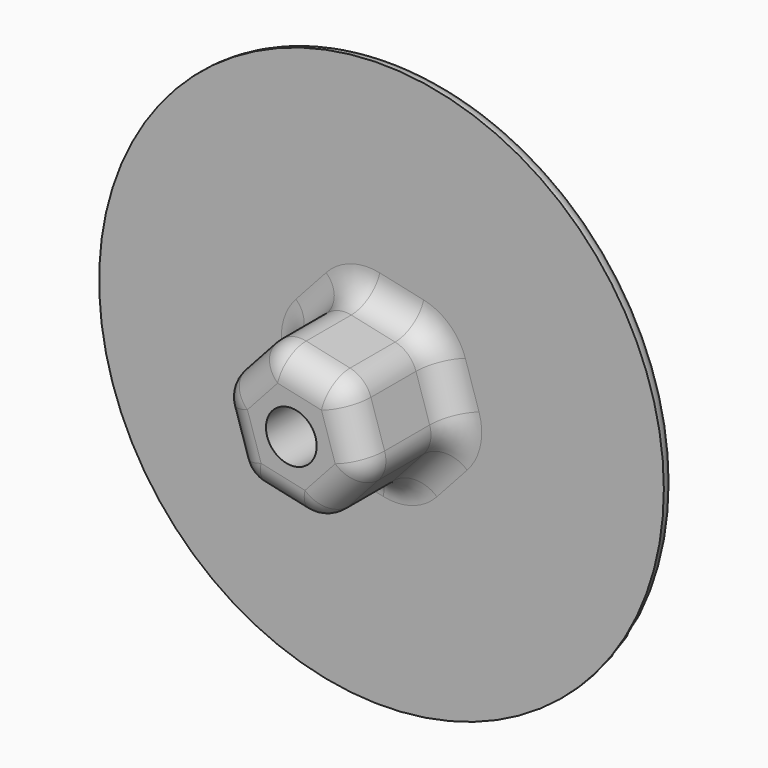
from build123d import *

# Parameters (mm, degrees)
F0_R     = 50.1
F0_R_2   = 4.5
F1_DEPTH = 3
F2_R     = 4.5
F3_DEPTH = 20
F4_R     = 2.99999
F5_R     = 5
F6_R     = 5


# Not quite as in the source:
# - a fillet or chamfer is up to 0.001 mm smaller than in the source, because OpenCascade refuses the exact size


with BuildPart() as f1:
    # F0 (on Front) → F1 (new body)
    with BuildSketch(Plane.XZ):
        Circle(F0_R)
        Circle(F0_R_2, mode=Mode.SUBTRACT)
    extrude(amount=F1_DEPTH)

    # F2 (on face) → F3 (join)
    with BuildSketch(Plane.XZ.offset(3)):
        Polygon((9.2398859849, 10.167053197), (-4.1849833578, 13.0855025895), (-13.4248693427, 2.9184493925), (-9.2398859849, -10.167053197), (4.1849833578, -13.0855025895), (13.4248693427, -2.9184493925), align=None)
        Circle(F2_R, mode=Mode.SUBTRACT)
    extrude(amount=F3_DEPTH)

    # F4 (radius 3 in the source; OpenCascade refuses exactly that, so slightly less here)
    f4_edges = [f1.edges().sort_by_distance(p)[0] for p in [
        (-50.1, 0, 0),
    ]]
    fillet(f4_edges, radius=F4_R)

    # F5
    f5_edges = [f1.edges().sort_by_distance(p)[0] for p in [
        (-4.184983, -13, 13.085503),
        (9.239886, -13, 10.167053),
        (13.424869, -13, -2.918449),
        (4.184983, -13, -13.085503),
        (-9.239886, -13, -10.167053),
        (-13.424869, -13, 2.918449),
    ]]
    fillet(f5_edges, radius=F5_R)

    # F6
    f6_edges = [f1.edges().sort_by_distance(p)[0] for p in [
        (11.332378, -3, 3.624302),
        (12.545511, -13, -0.168893),
        (10.119245, -13, 7.417497),
        (11.332378, -23, 3.624302),
    ]]
    fillet(f6_edges, radius=F6_R)


solid = f1.part
